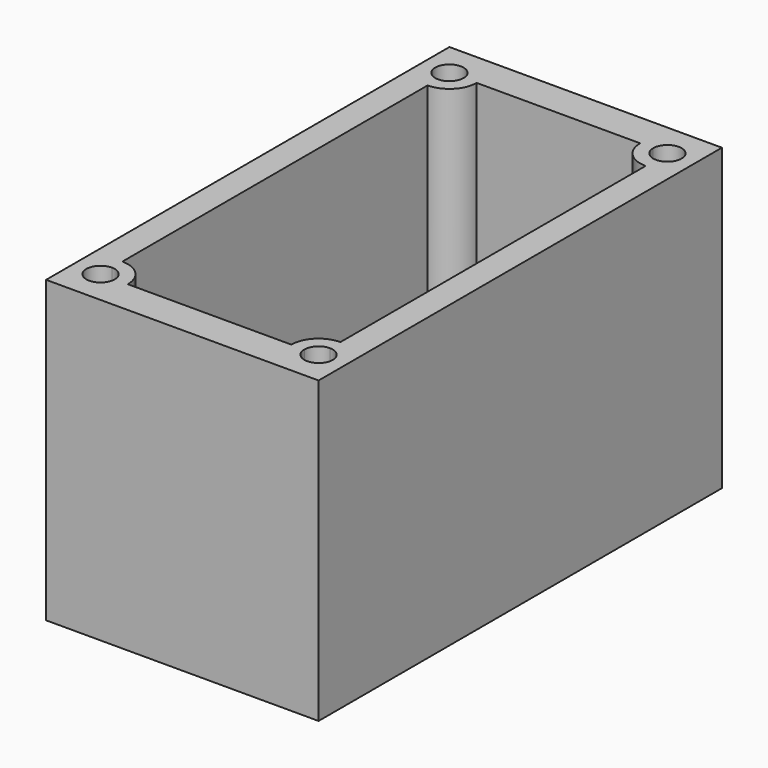
from build123d import *

# Parameters (mm, degrees)
F1_DEPTH = 34.925


with BuildPart() as f1:
    # F0 (on Top) → F1 (new body, symmetric)
    with BuildSketch(Plane.XY):
        with BuildLine():
            Line((-31.75, 50.8), (-31.75, -50.8))
            ThreePointArc((-31.75, -50.8), (-29.890128, -46.309872), (-25.4, -44.45))
            Line((-25.4, -44.45), (-25.4, 44.45))
            ThreePointArc((-25.4, 44.45), (-29.890128, 46.309872), (-31.75, 50.8))
        make_face()
        with BuildLine():
            ThreePointArc((19.05, 50.8), (25.4, 57.15), (31.75, 50.8))
            Line((31.75, 50.8), (31.75, 58.7375))
            Line((31.75, 58.7375), (-31.75, 58.7375))
            Line((-31.75, 58.7375), (-31.75, 50.8))
            ThreePointArc((-31.75, 50.8), (-25.4, 57.15), (-19.05, 50.8))
            Line((-19.05, 50.8), (19.05, 50.8))
        make_face()
        with BuildLine():
            ThreePointArc((-19.05, 50.8), (-25.4, 57.15), (-31.75, 50.8))
            ThreePointArc((-31.75, 50.8), (-29.890128, 46.309872), (-25.4, 44.45))
            Line((-25.4, 44.45), (-25.4, 47.498))
            ThreePointArc((-25.4, 47.498), (-27.734867, 53.134867), (-22.098, 50.8))
            Line((-22.098, 50.8), (-19.05, 50.8))
        make_face()
        with BuildLine():
            ThreePointArc((-25.4, 44.45), (-20.909872, 46.309872), (-19.05, 50.8))
            Line((-19.05, 50.8), (-22.098, 50.8))
            ThreePointArc((-22.098, 50.8), (-23.065133, 48.465133), (-25.4, 47.498))
            Line((-25.4, 47.498), (-25.4, 44.45))
        make_face()
        with BuildLine():
            ThreePointArc((-19.05, -50.8), (-20.909872, -46.309872), (-25.4, -44.45))
            Line((-25.4, -44.45), (-25.4, -47.498))
            ThreePointArc((-25.4, -47.498), (-23.065133, -48.465133), (-22.098, -50.8))
            Line((-22.098, -50.8), (-19.05, -50.8))
        make_face()
        with BuildLine():
            ThreePointArc((-25.4, -44.45), (-29.890128, -46.309872), (-31.75, -50.8))
            ThreePointArc((-31.75, -50.8), (-25.4, -57.15), (-19.05, -50.8))
            Line((-19.05, -50.8), (-22.098, -50.8))
            ThreePointArc((-22.098, -50.8), (-27.734867, -53.134867), (-25.4, -47.498))
            Line((-25.4, -47.498), (-25.4, -44.45))
        make_face()
        with BuildLine():
            Line((-31.75, -58.7375), (31.75, -58.7375))
            Line((31.75, -58.7375), (31.75, -50.8))
            ThreePointArc((31.75, -50.8), (25.4, -57.15), (19.05, -50.8))
            Line((19.05, -50.8), (-19.05, -50.8))
            ThreePointArc((-19.05, -50.8), (-25.4, -57.15), (-31.75, -50.8))
            Line((-31.75, -50.8), (-31.75, -58.7375))
        make_face()
        with BuildLine():
            ThreePointArc((19.05, -50.8), (25.4, -57.15), (31.75, -50.8))
            ThreePointArc((31.75, -50.8), (29.890128, -46.309872), (25.4, -44.45))
            Line((25.4, -44.45), (25.4, -47.498))
            ThreePointArc((25.4, -47.498), (27.734867, -48.465133), (28.702, -50.8))
            ThreePointArc((28.702, -50.8), (25.4, -54.102), (22.098, -50.8))
            Line((22.098, -50.8), (19.05, -50.8))
        make_face()
        with BuildLine():
            Line((25.4, -47.498), (25.4, -44.45))
            ThreePointArc((25.4, -44.45), (20.909872, -46.309872), (19.05, -50.8))
            Line((19.05, -50.8), (22.098, -50.8))
            ThreePointArc((22.098, -50.8), (23.065133, -48.465133), (25.4, -47.498))
        make_face()
        with BuildLine():
            ThreePointArc((25.4, 44.45), (29.890128, 46.309872), (31.75, 50.8))
            ThreePointArc((31.75, 50.8), (25.4, 57.15), (19.05, 50.8))
            Line((19.05, 50.8), (22.098, 50.8))
            ThreePointArc((22.098, 50.8), (25.4, 54.102), (28.702, 50.8))
            ThreePointArc((28.702, 50.8), (27.734867, 48.465133), (25.4, 47.498))
            Line((25.4, 47.498), (25.4, 44.45))
        make_face()
        with BuildLine():
            Line((22.098, 50.8), (19.05, 50.8))
            ThreePointArc((19.05, 50.8), (20.909872, 46.309872), (25.4, 44.45))
            Line((25.4, 44.45), (25.4, 47.498))
            ThreePointArc((25.4, 47.498), (23.065133, 48.465133), (22.098, 50.8))
        make_face()
        with BuildLine():
            ThreePointArc((25.4, -44.45), (29.890128, -46.309872), (31.75, -50.8))
            Line((31.75, -50.8), (31.75, 50.8))
            ThreePointArc((31.75, 50.8), (29.890128, 46.309872), (25.4, 44.45))
            Line((25.4, 44.45), (25.4, -44.45))
        make_face()
    extrude(amount=F1_DEPTH, both=True)


solid = f1.part
